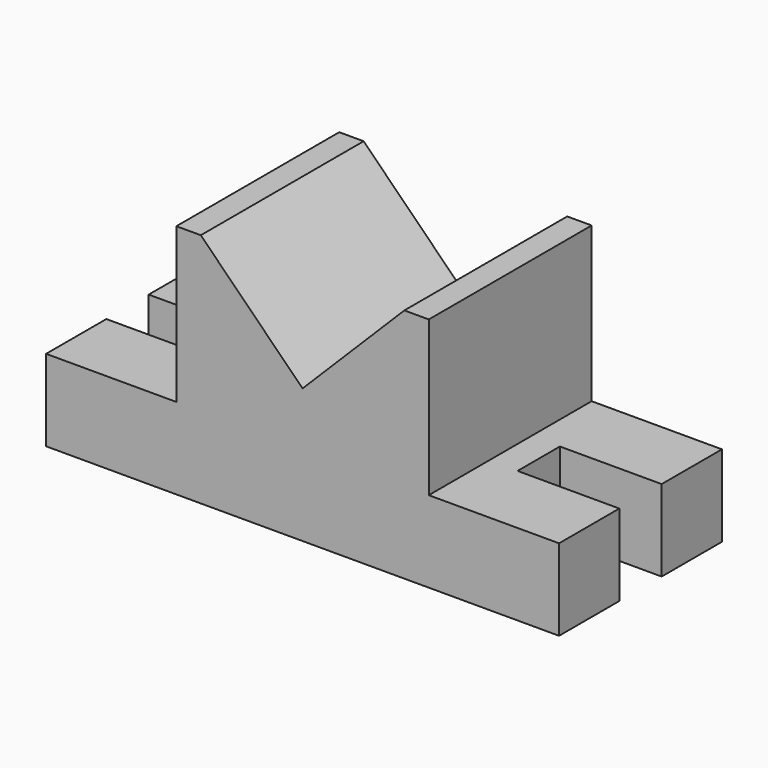
from build123d import *

# Parameters (mm, degrees)
F1_DEPTH = 50
F2_W     = 25
F2_H     = 13
F3_DEPTH = 20.001
F4_DEPTH = 20.001


# Not quite as in the source:
# - ends of sketch curves that miss each other by under 0.0002 mm in the source are joined


with BuildPart() as f1:
    # F0 (on Front) → F1 (new body)
    with BuildSketch(Plane.XZ):
        Polygon((-63, 0), (0, 0), (63, 0), (63, 20), (31, 20), (31, 58), (25, 58), (0, 32.9999986697), (-25.0000013303, 57.9999986697), (-31.0000013303, 57.9999986697), (-31.0000013303, 20), (-63.0000013303, 20), align=None)
    extrude(amount=F1_DEPTH)

    # F2 (on face) → F3 (cut, through all)
    with BuildSketch(Plane.XY.offset(20)):
        with Locations((-50.5000013303, -25)):
            Rectangle(F2_W, F2_H)
    extrude(amount=-F3_DEPTH, mode=Mode.SUBTRACT)

    # F2 (on face) → F4 (cut, through all)
    with BuildSketch(Plane.XY.offset(20)):
        with Locations((50.5000013303, -25)):
            Rectangle(F2_W, F2_H)
    extrude(amount=-F4_DEPTH, mode=Mode.SUBTRACT)


solid = f1.part
